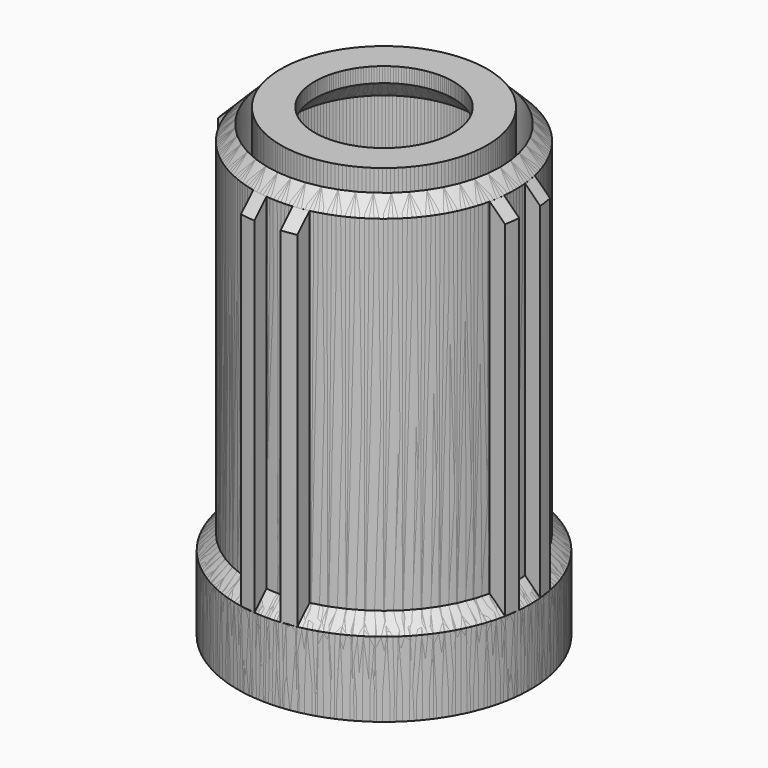
from build123d import *

# Parameters (mm, degrees)
F3_SIZE  = 1.99999
F6_DEPTH = 58
F7_SIZE  = 1.99999
F8_COUNT = 4


# Not quite as in the source:
# - a fillet or chamfer is up to 0.001 mm smaller than in the source, because OpenCascade refuses the exact size


with BuildPart() as f2:
    # F0 (on Right) → F2 (revolve)
    with BuildSketch(Plane.YZ):
        Polygon((-9.25, 0), (-9.25, 2), (-13.75, 2), (-13.75, -58), (-15.5, -58), (-15.5, 0), (-17.5, 0), (-17.5, -50), (-19.5, -50), (-19.5, -60), (-17.5, -60), (-12.25, -60), (-12.25, -3), (-12.25, 0), align=None)
        Polygon((-12.25, -3), (-9.25, 0), (-12.25, 0), align=None)
    revolve(axis=Axis((0, 0, 10.6590054929), (0, 0, -1)))

    # F3 (size 2 in the source; OpenCascade refuses exactly that, so slightly less here)
    f3_edges = [f2.edges().sort_by_distance(p)[0] for p in [
        (0, 17.5, 0),
        (0, 17.5, -50),
        (0, -17.5, -25),
    ]]
    chamfer(f3_edges, length=F3_SIZE)

    # F5 (on offset) → F6 (join)
    with BuildSketch(Plane(origin=(0, 0, -60), x_dir=(1, 0, 0), z_dir=(0, 0, -1))):
        with BuildLine():
            Line((-19.4213156094, 1.75), (-16.5, 1.75))
            Line((-16.5, 1.75), (-16.5, 3.75))
            Line((-16.5, 3.75), (-19.1360262333, 3.75))
            ThreePointArc((-19.1360262333, 3.75), (-19.3045888973, 2.7536970616), (-19.4213156094, 1.75))
        make_face()
        with BuildLine():
            Line((-16.5, -1.75), (-19.4213156094, -1.75))
            ThreePointArc((-19.4213156094, -1.75), (-19.3045888973, -2.7536970616), (-19.1360262333, -3.75))
            Line((-19.1360262333, -3.75), (-16.5, -3.75))
            Line((-16.5, -3.75), (-16.5, -1.75))
        make_face()
    extrude(amount=-F6_DEPTH)

    # F7 (size 2 in the source; OpenCascade refuses exactly that, so slightly less here)
    f7_edges = [f2.edges().sort_by_distance(p)[0] for p in [
        (-19.304589, -2.753697, -2),
        (-19.304589, 2.753697, -2),
    ]]
    chamfer(f7_edges, length=F7_SIZE)


with BuildPart() as f8_1:
    # F8: instance of F2
    add(f2.part.rotate(Axis((0, 0, 10.6590054929), (0, 0, -1)), 1 * 360 / F8_COUNT))


with BuildPart() as f8_2:
    # F8: instance of F2
    add(f2.part.rotate(Axis((0, 0, 10.6590054929), (0, 0, -1)), 2 * 360 / F8_COUNT))


with BuildPart() as f8_3:
    # F8: instance of F2
    add(f2.part.rotate(Axis((0, 0, 10.6590054929), (0, 0, -1)), 3 * 360 / F8_COUNT))


solid = Compound([f2.part, f8_1.part, f8_2.part, f8_3.part])
